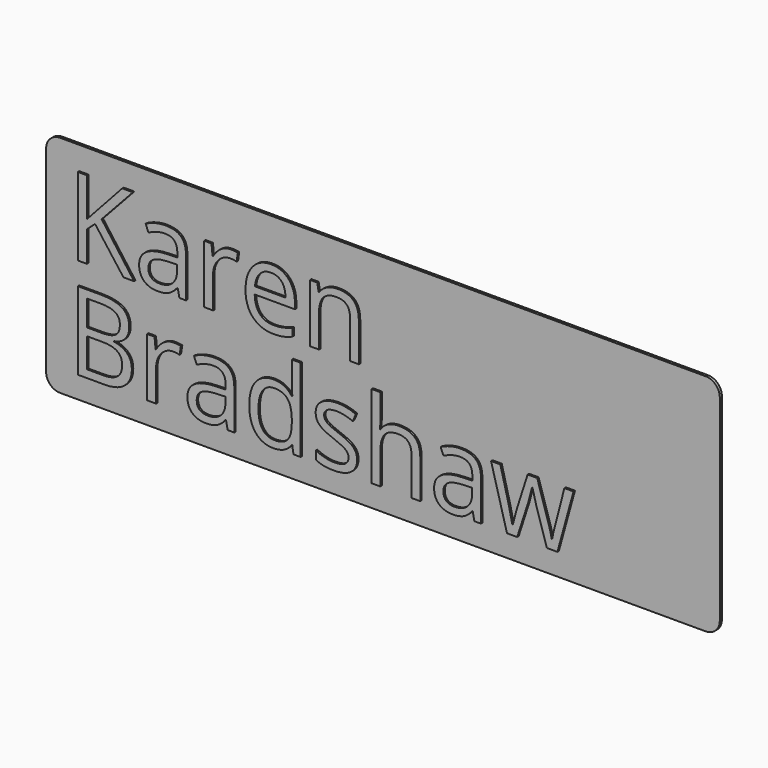
from build123d import *

# Parameters (mm, degrees)
F1_DEPTH     = 0.6
F2_TEXT_SIZE = 24.6944444444
F3_DEPTH     = 0.4


# Not quite as in the source:
# - Text() gives the source's letters only with a copy of the font that has no kerning and outlines rounded to 1/6400 em; it was checked with that copy


with BuildPart() as f1:
    # F0 (on Front) → F1 (new body)
    with BuildSketch(Plane.XZ):
        with BuildLine():
            Line((149.225, 0), (3.175, 0))
            ThreePointArc((3.175, 0), (0.9299359697, -0.9299359697), (0, -3.175))
            Line((0, -3.175), (0, -47.625))
            ThreePointArc((0, -47.625), (0.9299359697, -49.8700640303), (3.175, -50.8))
            Line((3.175, -50.8), (149.225, -50.8))
            ThreePointArc((149.225, -50.8), (151.4700640303, -49.8700640303), (152.4, -47.625))
            Line((152.4, -47.625), (152.4, -3.175))
            ThreePointArc((152.4, -3.175), (151.4700640303, -0.9299359697), (149.225, 0))
        make_face()
    extrude(amount=F1_DEPTH)

    # F2 (on face) → F3 (join)
    with BuildSketch(Plane.XZ.offset(0.6)):
        with Locations((5.08, -22.86)):
            Text('Karen', F2_TEXT_SIZE, font='Open Sans', text_align=(TextAlign.LEFT, TextAlign.BOTTOM))
        with Locations((5.08, -45.6102915394)):
            Text('Bradshaw', F2_TEXT_SIZE, font='Open Sans', text_align=(TextAlign.LEFT, TextAlign.BOTTOM))
    extrude(amount=F3_DEPTH)


solid = f1.part
